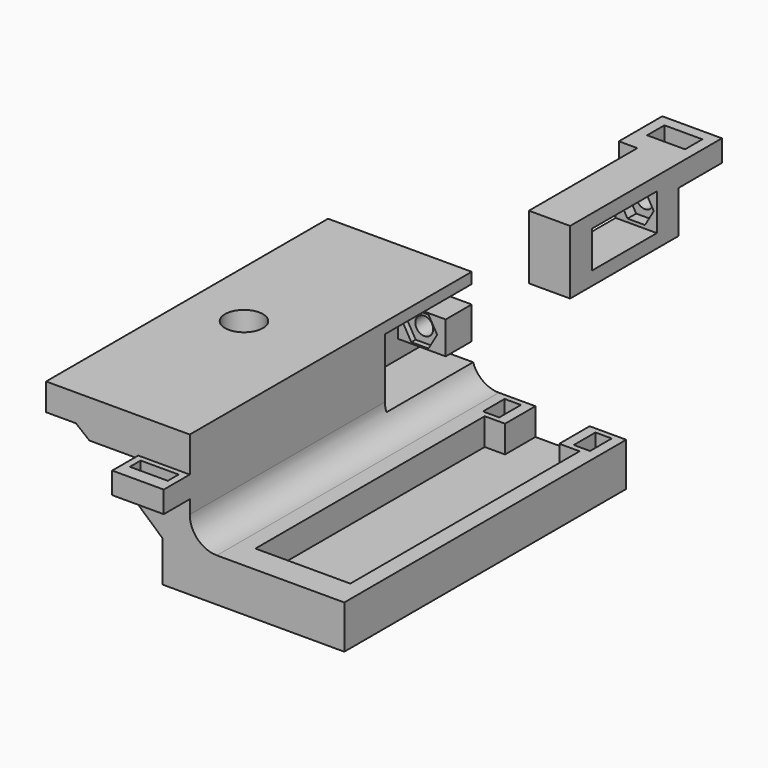
from build123d import *

# Parameters (mm, degrees)
F1_DEPTH  = 65
F2_R      = 3.5
F3_DEPTH  = 7
F5_DEPTH  = 5
F7_DEPTH  = 17.5
F9_W      = 6
F9_H      = 4
F10_DEPTH = 9.5
F11_W     = 7
F11_H     = 2.5
F12_DEPTH = 4
F15_DEPTH = 8
F16_R     = 1.65
F17_DEPTH = 6
F18_R     = 1.65
F19_DEPTH = 1
F20_DEPTH = 8
F21_DEPTH = 1.0139122871
F22_W     = 3
F22_H     = 5
F23_DEPTH = 8
F24_W     = 25
F24_H     = 11.8
F24_W_2   = 15
F24_H_2   = 6.8
F25_DEPTH = 7.6
F26_R     = 1.55
F27_DEPTH = 5
F28_R     = 1.55
F29_DEPTH = 2
F30_W     = 7
F30_H     = 4
F31_DEPTH = 4


# Not quite as in the source:
# - a feature names something its author has since deleted; it is built from what else it names


with BuildPart() as f1:
    # F0 (on Front) → F1 (new body)
    with BuildSketch(Plane.XZ):
        with BuildLine():
            Line((0, 26), (0, 21))
            Line((0, 21), (5.5, 21))
            Line((5.5, 21), (8, 19))
            Line((8, 19), (17, 19))
            Line((17, 19), (17, 11.5))
            Line((17, 11.5), (21.5, 7.5))
            Line((21.5, 7.5), (21.5, 0))
            Line((21.5, 0), (55, 0))
            Line((55, 0), (55, 8))
            Line((55, 8), (31.5, 8))
            ThreePointArc((31.5, 8), (27.9644660941, 9.4644660941), (26.5, 13))
            Line((26.5, 13), (26.5, 26))
            Line((26.5, 26), (0, 26))
        make_face()
    extrude(amount=F1_DEPTH)

    # F2 (on face) → F3 (cut, through all)
    with BuildSketch(Plane.XY.offset(26)):
        with Locations((10.5, -32.5)):
            Circle(F2_R)
    extrude(amount=-F3_DEPTH, mode=Mode.SUBTRACT)

    # F4 (on face) → F5 (cut)
    with BuildSketch(Plane.XY.offset(8)):
        Polygon((34.5, -62), (52, -62), (52, -7), (48.25, -7), (48.25, 0), (38.25, 0), (38.25, -7), (34.5, -7), align=None)
    extrude(amount=-F5_DEPTH, mode=Mode.SUBTRACT)

    # F6 (on face) → F7 (join, through all)
    with BuildSketch(Plane.YZ.offset(34.5)):
        Polygon((-62, 8), (-62, 4.2981612496), (-59.862742401, 8), align=None)
    extrude(amount=F7_DEPTH)

    # F9 (on offset) → F10 (join, through all)
    with BuildSketch(Plane.YZ.offset(26.5)):
        with Locations((-68, 17.5)):
            Rectangle(F9_W, F9_H)
    extrude(amount=-F10_DEPTH)

    # F11 (on face) → F12 (cut, through all)
    with BuildSketch(Plane.XY.offset(19.5)):
        with Locations((21.75, -67.25)):
            Rectangle(F11_W, F11_H)
    extrude(amount=-F12_DEPTH, mode=Mode.SUBTRACT)

    # F14 (on offset) → F15 (cut)
    with BuildSketch(Plane.YZ.offset(25.75)):
        Polygon((-20, 11.4), (0, 11.4), (0, 14.7), (-6, 14.7), (-6, 20.7), (0, 20.7), (0, 24), (-20, 24), align=None)
    extrude(amount=-F15_DEPTH, mode=Mode.SUBTRACT)

    # F16 (on face) → F17 (cut, through all)
    with BuildSketch(Plane(origin=(0, 0, 0), x_dir=(-1, 0, 0), z_dir=(0, 1, 0))):
        with Locations((-21.75, 17.7)):
            Circle(F16_R)
    extrude(amount=-F17_DEPTH, mode=Mode.SUBTRACT)

    # F18 (on face) → F19 (cut)
    with BuildSketch(Plane.XZ.offset(6)):
        Polygon((23.3377132403, 14.95), (24.9254264805, 17.7), (23.3377132403, 20.45), (20.1622867597, 20.45), (18.5745735195, 17.7), (20.1622867597, 14.95), align=None)
        with Locations((21.75, 17.7)):
            Circle(F18_R, mode=Mode.SUBTRACT)
    extrude(amount=-F19_DEPTH, mode=Mode.SUBTRACT)

    # F14 (on offset) → F20 (cut, through all)
    with BuildSketch(Plane.YZ.offset(25.75)):
        Polygon((-20, 11.4), (0, 11.4), (0, 14.7), (-6, 14.7), (-6, 20.7), (0, 20.7), (0, 24), (-20, 24), align=None)
    extrude(amount=-F20_DEPTH, mode=Mode.SUBTRACT)

    # F14 (on offset) → F21 (cut, through all)
    with BuildSketch(Plane.YZ.offset(25.75)):
        Polygon((-20, 11.4), (0, 11.4), (0, 14.7), (-6, 14.7), (-6, 20.7), (0, 20.7), (0, 24), (-20, 24), align=None)
    extrude(amount=F21_DEPTH, mode=Mode.SUBTRACT)

    # F22 (on face) → F23 (cut, through all)
    with BuildSketch(Plane.XY.offset(8)):
        with Locations((34.875, -3.5)):
            Rectangle(F22_W, F22_H)
        with Locations((51.625, -3.5)):
            Rectangle(F22_W, F22_H)
    extrude(amount=-F23_DEPTH, mode=Mode.SUBTRACT)


with BuildPart() as f25:
    # F24 (on offset) → F25 (new body)
    with BuildSketch(Plane.YZ.offset(25.75)):
        with Locations((36.1234692893, 17.7)):
            Rectangle(F24_W, F24_H)
        with Locations((36.1234692893, 17.7)):
            Rectangle(F24_W_2, F24_H_2, mode=Mode.SUBTRACT)
    extrude(amount=-F25_DEPTH)

    # F26 (on face) → F27 (cut, through all)
    with BuildSketch(Plane(origin=(0, 48.6234692893, 0), x_dir=(-1, 0, 0), z_dir=(0, 1, 0))):
        with Locations((-21.95, 17.7)):
            Circle(F26_R)
    extrude(amount=-F27_DEPTH, mode=Mode.SUBTRACT)

    # F28 (on face) → F29 (cut)
    with BuildSketch(Plane.XZ.offset(-43.6234692893)):
        Polygon((23.5665807537, 14.9), (25.1831615075, 17.7), (23.5665807537, 20.5), (20.3334192463, 20.5), (18.7168384925, 17.7), (20.3334192463, 14.9), align=None)
        with Locations((21.95, 17.7)):
            Circle(F28_R, mode=Mode.SUBTRACT)
    extrude(amount=-F29_DEPTH, mode=Mode.SUBTRACT)

    # F30 (on face) → F31 (join)
    with BuildSketch(Plane.XY.offset(23.6)):
        Polygon((14.75, 58.6234692893), (14.75, 48.6234692893), (18.15, 48.6234692893), (25.75, 48.6234692893), (25.75, 58.6234692893), align=None)
        with Locations((20.25, 54.6234692893)):
            Rectangle(F30_W, F30_H, mode=Mode.SUBTRACT)
    extrude(amount=-F31_DEPTH)


solid = Compound([f1.part, f25.part])
